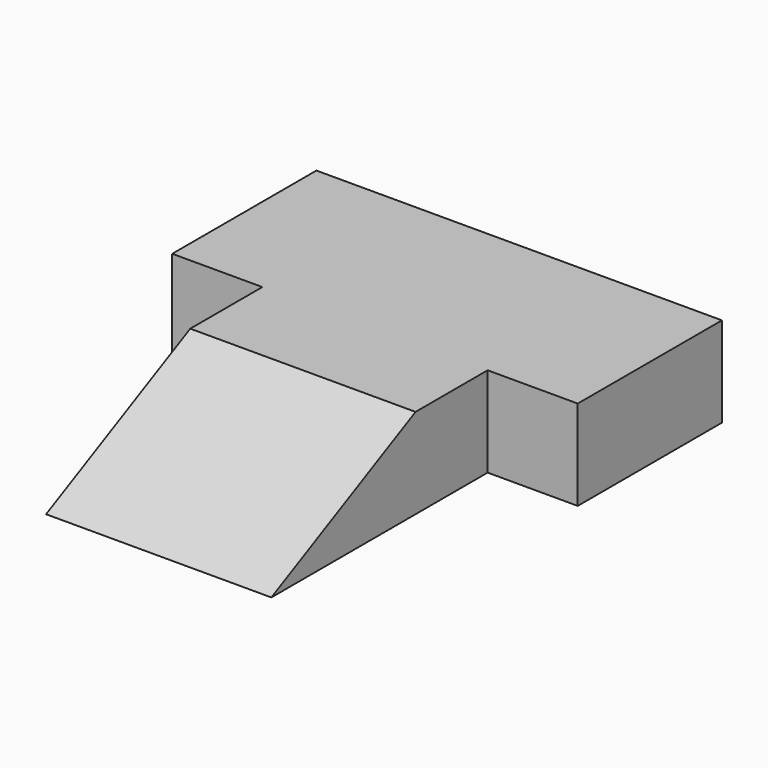
from build123d import *

# Parameters (mm, degrees)
F0_W     = 50
F0_H     = 20
F1_DEPTH = 100
F2_SIZE2 = 39.99999
F2_SIZE  = 19.99999
F3_W     = 40
F3_H     = 20
F4_DEPTH = 20
F5_W     = 40
F5_H     = 20
F6_DEPTH = 20


# Not quite as in the source:
# - a fillet or chamfer is up to 0.001 mm smaller than in the source, because OpenCascade refuses the exact size


with BuildPart() as f1:
    # F0 (on Front) → F1 (new body)
    with BuildSketch(Plane.XZ):
        Rectangle(F0_W, F0_H)
    extrude(amount=F1_DEPTH)

    # F2 (size 20 and 40 in the source; OpenCascade refuses exactly that, so slightly less here)
    f2_edges = [f1.edges().sort_by_distance(p)[0] for p in [
        (0, -100, 10),
    ]]
    f2_side = f1.faces().sort_by_distance((0, -100, 0))[0]
    chamfer(f2_edges, length=F2_SIZE, length2=F2_SIZE2, reference=f2_side)

    # F3 (on face) → F4 (join)
    with BuildSketch(Plane.YZ.offset(25)):
        with Locations((-20, 0)):
            Rectangle(F3_W, F3_H)
    extrude(amount=F4_DEPTH)

    # F5 (on face) → F6 (join)
    with BuildSketch(Plane(origin=(-25, 0, 0), x_dir=(0, -1, 0), z_dir=(-1, 0, 0))):
        with Locations((20, 0)):
            Rectangle(F5_W, F5_H)
    extrude(amount=F6_DEPTH)


solid = f1.part
